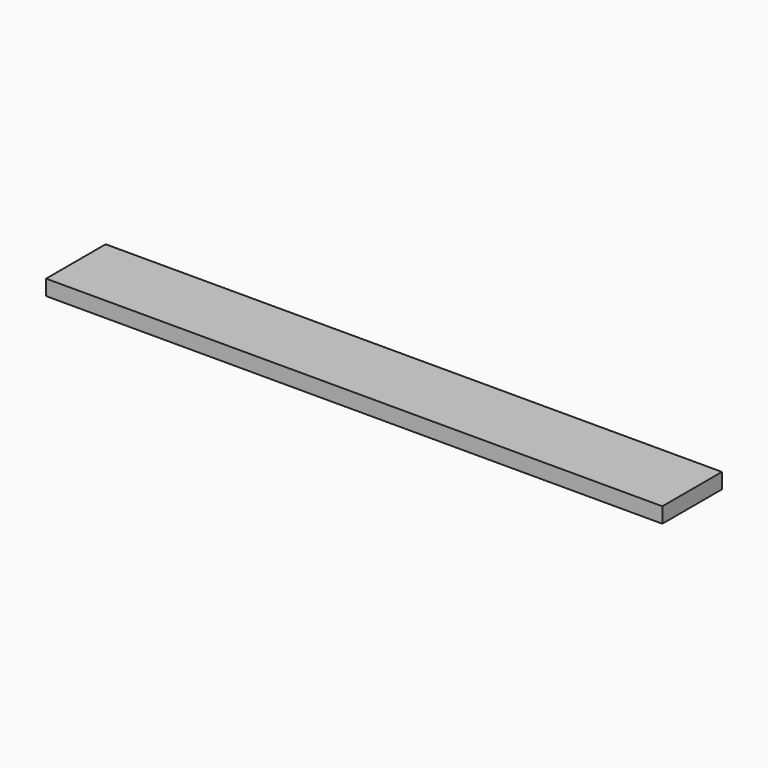
from build123d import *

# Parameters (mm, degrees)
F1_W     = 184.15
F1_H     = 38.1
F2_DEPTH = 762


# Not quite as in the source:
# - a variable given as a bare number and used for a length is read in inches; the dataset says mm whatever the document's units were


with BuildPart() as f2:
    # F1 (on Right) → F2 (new body, symmetric)
    with BuildSketch(Plane.YZ):
        Rectangle(F1_W, F1_H)
    extrude(amount=F2_DEPTH, both=True)


solid = f2.part
